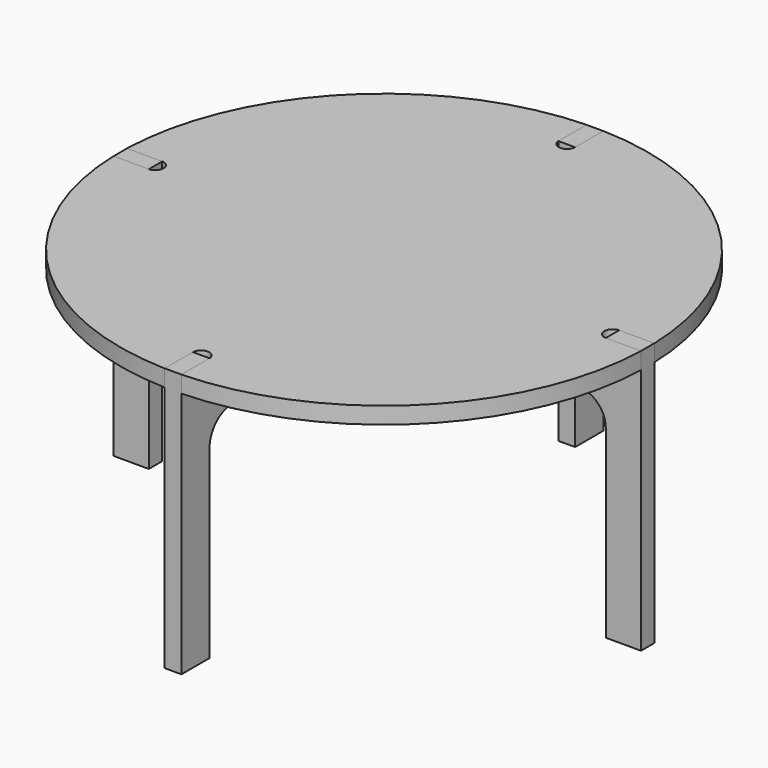
from build123d import *

# Parameters (mm, degrees)
F0_R            = 300
F1_DEPTH        = 19
F3_DEPTH        = 9.5
F3_DEPTH_BACK   = 9.5
F4_R            = 31
F4_2_R          = 31
F8_DEPTH        = 300.001
F8_COPIES_COUNT = 4


# Not quite as in the source:
# - a feature of the source that left no trace in its solid (it failed there, or was rolled back) is left out
# - a pattern or mirror of a feature is missing from the dataset's text; its kind, count and spacing are read off the source's solid


with BuildPart() as f1:
    # F0 (on Top) → F1 (new body)
    with BuildSketch(Plane.XY):
        Circle(F0_R)
    extrude(amount=F1_DEPTH)

    # F7 (on face) → F8 (cut, through all)
    with BuildSketch(Plane.XY.offset(19)):
        with BuildLine():
            Line((-340, -9.5), (-260, -9.5))
            ThreePointArc((-260, -9.5), (-250.5, 0), (-260, 9.5))
            Line((-260, 9.5), (-340, 9.5))
            Line((-340, 9.5), (-340, -9.5))
        make_face()
    f8 = extrude(amount=-F8_DEPTH, mode=Mode.SUBTRACT)

    # F8_copies: F8 ×4 about axis
    f8_copies_axis = Axis((0, 0, 0), (0, 0, 1))
    for i in range(1, F8_COPIES_COUNT):
        add(f8.rotate(f8_copies_axis, i * 360 / F8_COPIES_COUNT), mode=Mode.SUBTRACT)


with BuildPart() as f3:
    # F2 (on Front) → F3 (new body, two sides)
    with BuildSketch(Plane.XZ) as f3_sk:
        Polygon((-259.7109091582, 19), (-299.7109091582, 19), (-299.7109091582, -281), (-259.7109091582, -281), (-259.7109091582, -40), (0, -40), (0, 0), (-259.7109091582, 0), align=None)
        Polygon((259.7109091582, 0), (0, 0), (0, -40), (259.7109091582, -40), (259.7109091582, -281), (299.7109091582, -281), (299.7109091582, 19), (259.7109091582, 19), align=None)
    extrude(amount=F3_DEPTH)
    extrude(f3_sk.sketch, amount=-F3_DEPTH_BACK)


with BuildPart() as f3_copies_1:
    # F3_copies: instance of F3
    add(f3.part.mirror(Plane(origin=(0, 0, 0), x_dir=(0.7071067812, 0.7071067812, 0), z_dir=(-0.7071067812, 0.7071067812, 0))))

    # F4#2
    f4_2_edges = [f3_copies_1.edges().sort_by_distance(p)[0] for p in [
        (0, -259.710909, -40),
        (0, 259.710909, -40),
    ]]
    fillet(f4_2_edges, radius=F4_2_R)


with BuildPart() as f3_1:
    add(f3.part)

    # F4
    f4_edges = [f3_1.edges().sort_by_distance(p)[0] for p in [
        (-259.710909, 0, -40),
        (259.710909, 0, -40),
    ]]
    fillet(f4_edges, radius=F4_R)


solid = Compound([f1.part, f3_copies_1.part, f3_1.part])
